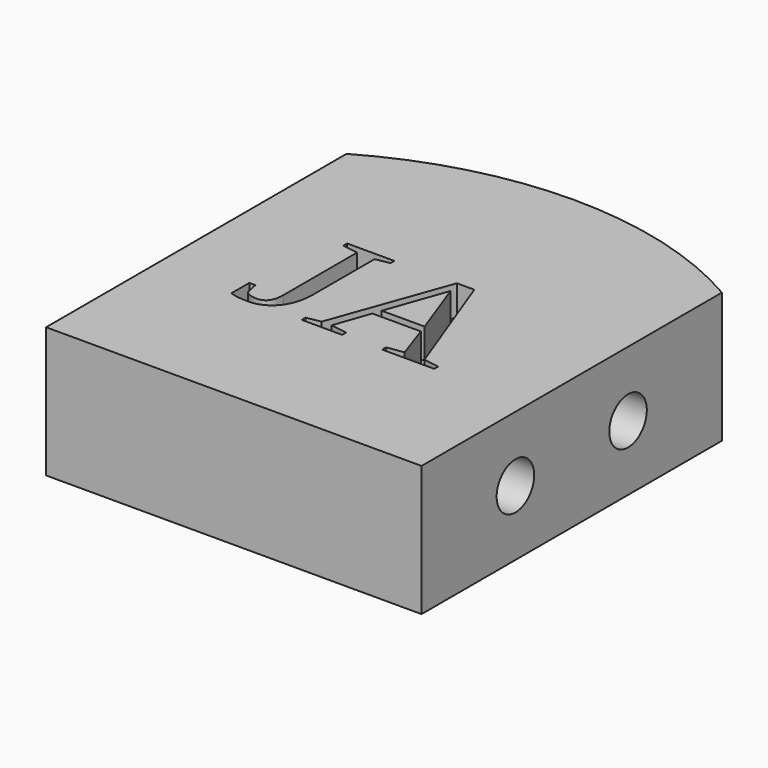
from build123d import *

# Parameters (mm, degrees)
F0_W         = 40
F0_H         = 40
F1_DEPTH     = 13.9
F2_R         = 2.5
F3_DEPTH     = 50
F4_TEXT_SIZE = 20.0209207833
F5_DEPTH     = 3.2


# Not quite as in the source:
# - Text() gives the source's letters only with a copy of the font that has no kerning and outlines rounded to 1/6400 em; it was checked with that copy


with BuildPart() as f1:
    # F0 (on Top) → F1 (new body)
    with BuildSketch(Plane.XY):
        with Locations((-2.9836571962, -27.5411564112)):
            Rectangle(F0_W, F0_H)
        with BuildLine():
            Line((-22.9836571962, -7.5411564112), (17.0163428038, -7.5411564112))
            ThreePointArc((17.0163428038, -7.5411564112), (-2.9836571962, -2.1821725625), (-22.9836571962, -7.5411564112))
        make_face()
    extrude(amount=F1_DEPTH)

    # F2 (on face) → F3 (cut)
    with BuildSketch(Plane(origin=(-22.9836571962, 0, 0), x_dir=(0, -1, 0), z_dir=(-1, 0, 0))):
        with Locations((20.0411564112, 6.95)):
            Circle(F2_R)
        with Locations((35.0411564112, 6.95)):
            Circle(F2_R)
    extrude(amount=-F3_DEPTH, mode=Mode.SUBTRACT)

    # F4 (on face) → F5 (cut)
    with BuildSketch(Plane.XY.offset(13.9)):
        with Locations((-15.1916031027, -33.2212578505)):
            Text('JA', F4_TEXT_SIZE, font='Tinos', text_align=(TextAlign.LEFT, TextAlign.BOTTOM))
    extrude(amount=-F5_DEPTH, mode=Mode.SUBTRACT)


solid = f1.part
